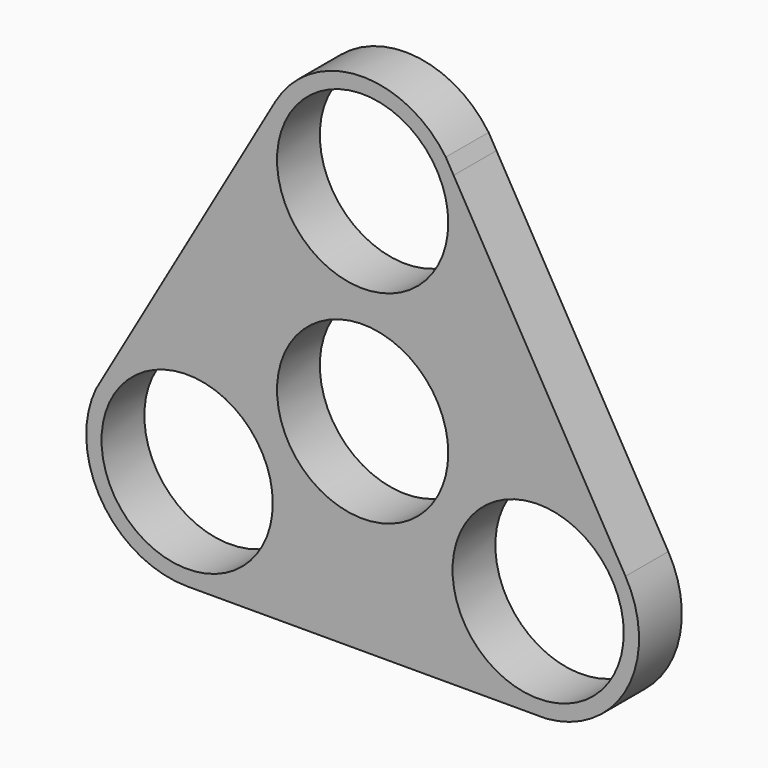
from build123d import *

# Parameters (mm, degrees)
F0_R     = 11.2
F1_DEPTH = 7


# Not quite as in the source:
# - ends of sketch curves that miss each other by under 0.0002 mm in the source are joined


with BuildPart() as f1:
    # F0 (on Front) → F1 (new body)
    with BuildSketch(Plane.XZ):
        with BuildLine():
            Line((34.3850237921, -6.6456524925), (11.9034600857, 32.216063506))
            Line((11.9034600857, 32.216063506), (10.8795652547, 33.9859719811))
            ThreePointArc((10.8795652547, 33.9859719811), (-0.5229512338, 39.7006466997), (-11.4372271683, 33.1011413973))
            ThreePointArc((-11.4372271683, 33.1011413973), (-11.443253047, 33.0906723652), (-11.449269343, 33.0801978231))
            Line((-11.449269343, 33.0801978231), (-33.8515173907, -5.7990863826))
            Line((-33.8515173907, -5.7990863826), (-34.8724977352, -7.5710060978))
            ThreePointArc((-34.8724977352, -7.5710060978), (-34.1203065589, -20.3032101841), (-22.9478157697, -26.4554889214))
            ThreePointArc((-22.9478157697, -26.4554889214), (-22.9392839252, -26.4554787883), (-22.930752089, -26.4554631407))
            Line((-22.930752089, -26.4554631407), (21.9480379364, -26.4167307195))
            Line((21.9480379364, -26.4167307195), (23.9929324806, -26.4149658832))
            ThreePointArc((23.9929324806, -26.4149658832), (34.6432297092, -19.3974365399), (34.3850237921, -6.6456524925))
        make_face()
        with Locations((-22.9592271072, -13.2554938539)):
            Circle(F0_R, mode=Mode.SUBTRACT)
        with Locations((22.9591888153, -13.2555159617)):
            Circle(F0_R, mode=Mode.SUBTRACT)
        Circle(F0_R, mode=Mode.SUBTRACT)
        with Locations((0, 26.5110097826)):
            Circle(F0_R, mode=Mode.SUBTRACT)
    extrude(amount=F1_DEPTH)


solid = f1.part
